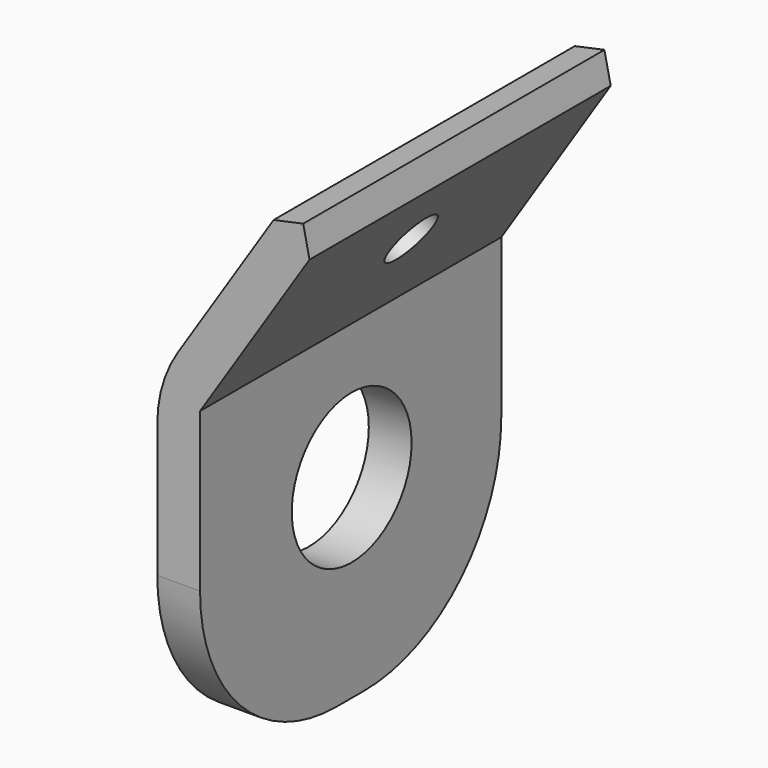
from build123d import *

# Parameters (mm, degrees)
F1_DEPTH    = 44
F2_R        = 15
F3_T1_DEPTH = 69.7168298797
F4_R        = 20
F5_R        = 8.75
F6_DEPTH    = 25
F7_R        = 3.25
F8_DEPTH    = 25


# Not quite as in the source:
# - a fillet or chamfer that OpenCascade refuses, or shapes differently, is made with other operations: its cross-section is extruded or revolved along the edge and cut away or added


with BuildPart() as f1:
    # F0 (on Front) → F1 (new body)
    with BuildSketch(Plane.XZ):
        Polygon((29.4669866014, 53.6632488984), (13.1538538262, 28.4862415493), (13.1538538262, -11.5137584507), (18.1538538262, -11.5137584507), (18.1538538262, 27.0079869683), (33.6631544929, 50.9443934359), align=None)
    extrude(amount=F1_DEPTH)

    # F2
    f2_edges = [f1.edges().sort_by_distance(p)[0] for p in [
        (13.153854, -22, 28.486242),
    ]]
    fillet(f2_edges, radius=F2_R)

    # F3: chamfer of 5 on 2 edges, made by hand

    # F3_s2 → F3_t1 (cut)
    with BuildSketch(Plane.XZ.offset(-12.8584149398)):
        Polygon((26.7481311389, 49.4670810069), (33.6631544929, 50.9443934359), (29.4669866014, 53.6632488984), align=None)
        Polygon((29.4669866014, 53.6632488984), (30.9442990304, 46.7482255444), (33.6631544929, 50.9443934359), align=None)
    extrude(amount=F3_T1_DEPTH, mode=Mode.SUBTRACT)

    # F4
    f4_edges = [f1.edges().sort_by_distance(p)[0] for p in [
        (15.653854, -44, -11.513758),
        (15.653854, 0, -11.513758),
    ]]
    fillet(f4_edges, radius=F4_R)

    # F5 (on face) → F6 (cut)
    with BuildSketch(Plane.YZ.offset(18.1538538262)):
        with Locations((-21.8509025872, 11.1763291061)):
            Circle(F5_R)
    extrude(amount=-F6_DEPTH, mode=Mode.SUBTRACT)

    # F7 (on face) → F8 (cut)
    with BuildSketch(Plane(origin=(0.4608744572, 0, -0.2986179457), x_dir=(0, 1, 0), z_dir=(0.8392335783, 0, -0.5437710925))):
        with Locations((-22.313432768, 45.9909811616)):
            Circle(F7_R)
    extrude(amount=-F8_DEPTH, mode=Mode.SUBTRACT)


solid = f1.part
